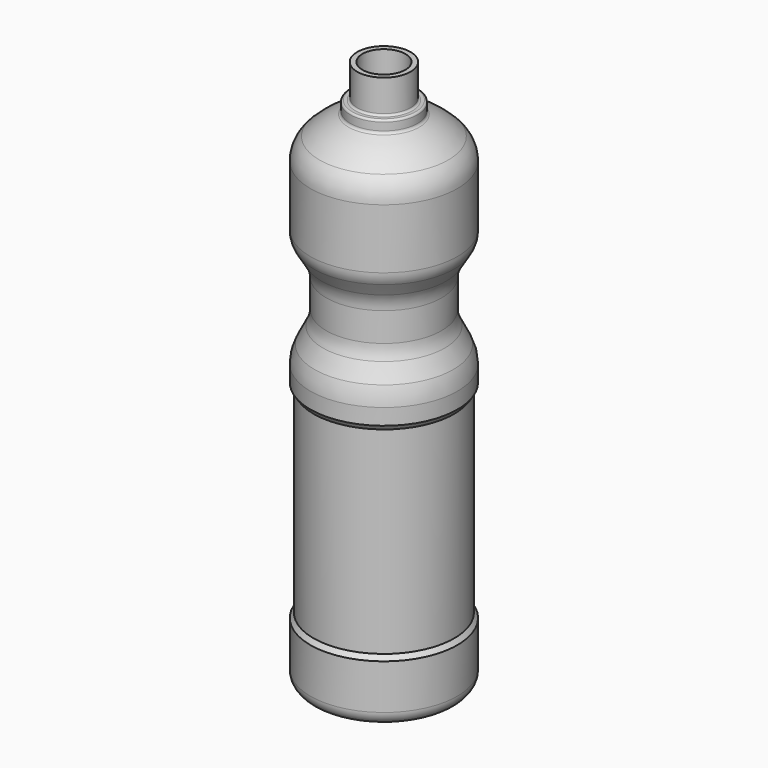
from build123d import *


# Not quite as in the source:
# - ends of sketch curves that miss each other by under 0.0002 mm in the source are joined


with BuildPart() as f3:
    # F2 (on Front) → F3 (revolve)
    with BuildSketch(Plane.XZ):
        with BuildLine():
            Line((7.8, 124.5), (7.8, 140.1))
            Line((7.8, 140.1), (5.145, 140.1))
            Line((5.145, 140.1), (5.145, 123.9))
            ThreePointArc((5.145, 123.9), (4.8521067812, 123.1928932188), (4.145, 122.9))
            Line((4.145, 122.9), (2.6, 122.9))
            ThreePointArc((2.6, 122.9), (1.8928932188, 122.6071067812), (1.6, 121.9))
            Line((1.6, 121.9), (1.6, 117.976082))
            ThreePointArc((1.6, 117.976082), (1.350130078, 117.1471219357), (0.6837669492, 116.5943381203))
            ThreePointArc((0.6837669492, 116.5943381203), (-7.1959862725, 112.3291290083), (-14.1126025069, 106.633258507))
            ThreePointArc((-14.1126025069, 106.633258507), (-17.5817732211, 101.4421014399), (-18.8, 95.318444))
            Line((-18.8, 95.318444), (-18.8, 64.723807))
            ThreePointArc((-18.8, 64.723807), (-18.3645791385, 61.5206040173), (-17.0899151086, 58.5498579349))
            Line((-17.0899151086, 58.5498579349), (-12.980113, 51.700188))
            ThreePointArc((-12.980113, 51.700188), (-11.2805611257, 47.7391932277), (-10.7, 43.468256))
            Line((-10.7, 43.468256), (-10.7, 28.719236))
            ThreePointArc((-10.7, 28.719236), (-11.1372317464, 25.0043679965), (-12.4250305354, 21.4925322711))
            Line((-12.4250305354, 21.4925322711), (-16.643712, 13.159334))
            ThreePointArc((-16.643712, 13.159334), (-18.2534603944, 8.7695396803), (-18.8, 4.125955))
            Line((-18.8, 4.125955), (-18.8, -4.1))
            Line((-18.8, -4.1), (-17.176481, -6.6))
            Line((-17.176481, -6.6), (-17.176481, -107.6))
            Line((-17.176481, -107.6), (-18.8, -110.1))
            Line((-18.8, -110.1), (-18.8, -133.1))
            ThreePointArc((-18.8, -133.1), (-16.7497474683, -138.0497474683), (-11.8, -140.1))
            Line((-11.8, -140.1), (-9.3, -140.1))
            ThreePointArc((-9.3, -140.1), (3.3189642091, -137.297082839), (16.1930179947, -136.133750794))
            ThreePointArc((16.1930179947, -136.133750794), (17.4098568229, -136.850666867), (18.8, -137.1))
            Line((18.8, -137.1), (18.8, -135.1))
            ThreePointArc((18.8, -135.1), (4.538075165, -136.1049653041), (-9.4419900149, -139.1))
            Line((-9.4419900149, -139.1), (-12.4, -139.1))
            ThreePointArc((-12.4, -139.1), (-16.6426406871, -137.3426406871), (-18.4, -133.1))
            Line((-18.4, -133.1), (-18.4, -110.218485399))
            Line((-18.4, -110.218485399), (-16.776481, -107.718485399))
            Line((-16.776481, -107.718485399), (-16.776481, -6.481514601))
            Line((-16.776481, -6.481514601), (-18.4, -3.981514601))
            Line((-18.4, -3.981514601), (-18.4, 4.125955))
            ThreePointArc((-18.4, 4.125955), (-17.8643911865, 8.6766679867), (-16.286837889, 12.9786664853))
            Line((-16.286837889, 12.9786664853), (-12.0681557678, 21.311864398))
            ThreePointArc((-12.0681557678, 21.311864398), (-10.74816254, 24.9114962964), (-10.3, 28.719236))
            Line((-10.3, 28.719236), (-10.3, 43.468256))
            ThreePointArc((-10.3, 43.468256), (-10.8950751539, 47.8459666584), (-12.6371159279, 51.9059862383))
            Line((-12.6371159279, 51.9059862383), (-16.7469178297, 58.7556563022))
            ThreePointArc((-16.7469178297, 58.7556563022), (-17.9790931672, 61.62737745), (-18.4, 64.723807))
            Line((-18.4, 64.723807), (-18.4, 95.318444))
            ThreePointArc((-18.4, 95.318444), (-17.2122288905, 101.2890100039), (-13.8297873838, 106.3503880838))
            ThreePointArc((-13.8297873838, 106.3503880838), (-6.9726050801, 111.9973145378), (0.8394378344, 116.2258737751))
            ThreePointArc((0.8394378344, 116.2258737751), (1.6834980988, 116.9260659186), (2, 117.976082))
            Line((2, 117.976082), (2, 121.9))
            ThreePointArc((2, 121.9), (2.1757359313, 122.3242640687), (2.6, 122.5))
            Line((2.6, 122.5), (5.8, 122.5))
            ThreePointArc((5.8, 122.5), (7.2142135624, 123.0857864376), (7.8, 124.5))
        make_face()
    revolve(axis=Axis((18.8, 0, -135.1), (0, 0, -1)))


with BuildPart() as f6:
    # F5 (on Front) → F6 (revolve)
    with BuildSketch(Plane.XZ):
        with BuildLine():
            Line((7.8, 124.4), (7.8, 140.1))
            Line((7.8, 140.1), (5.145, 140.1))
            Line((5.145, 140.1), (5.145, 122.9))
            Line((5.145, 122.9), (5.0757636953, 122.9))
            Line((5.0757636953, 122.9), (7.0503184624, 9.7778331549))
            ThreePointArc((7.0503184624, 9.7778331549), (9.1428874784, 4.9072468559), (14.0492523285, 2.9))
            Line((14.0492523285, 2.9), (17.5625566824, 2.9))
            Line((17.5625566824, 2.9), (18, -2.1))
            Line((18, -2.1), (18.8, -2.1))
            Line((18.8, -2.1), (18.8, 4.9))
            Line((18.8, 4.9), (14.7993665745, 4.9))
            ThreePointArc((14.7993665745, 4.9), (11.294820253, 6.3337477542), (9.8001280987, 9.8127379678))
            Line((9.8001280987, 9.8127379678), (7.8, 124.4))
        make_face()
    revolve(axis=Axis((18.8, 0, 1.4), (0, 0, -1)))


solid = Compound([f3.part, f6.part])
